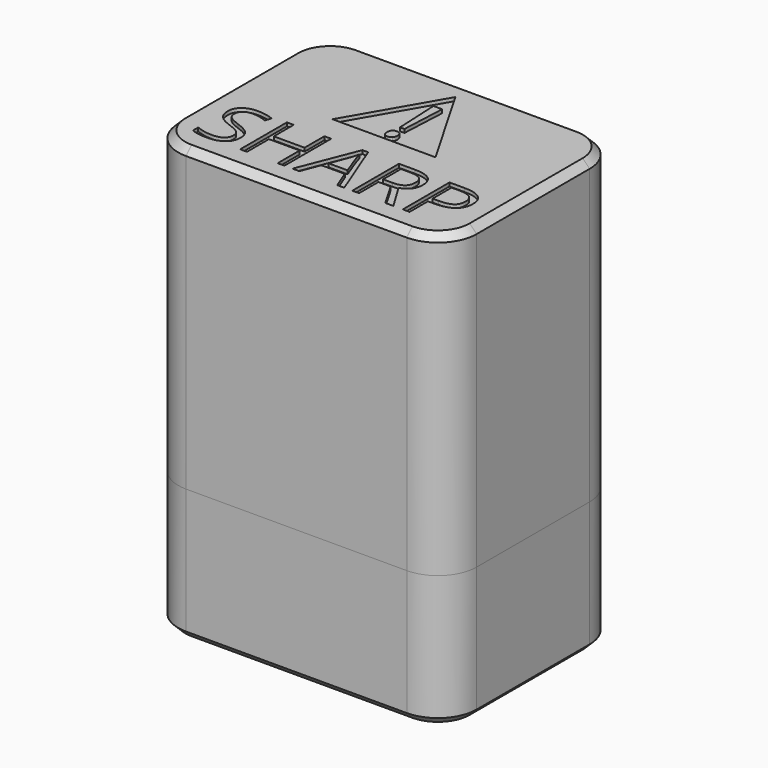
from build123d import *

# Parameters (mm, degrees)
F1_W          = 22
F1_H          = 43
F2_DEPTH      = 0.5
F4_DEPTH      = 37
F5_T          = 1.6
F7_DEPTH      = 15
F9_DEPTH      = 32
F11_DEPTH     = 2
F12_SIZE      = 0.8
F12_2_SIZE    = 0.8
F13_TEXT_SIZE = 9.2601952331
F14_DEPTH     = 0.4


# Not quite as in the source:
# - Text() gives the source's letters only with a copy of the font that has no kerning and outlines rounded to 1/6400 em; it was checked with that copy


with BuildPart() as f2:
    # F1 (on Front) → F2 (new body)
    with BuildSketch(Plane.XZ):
        with Locations((0, 21.5)):
            Rectangle(F1_W, F1_H)
    extrude(amount=F2_DEPTH)


with BuildPart() as f4:
    # F3 (on Top) → F4 (new body)
    with BuildSketch(Plane.XY):
        with BuildLine():
            Line((-12.5, -9), (12.5, -9))
            ThreePointArc((12.5, -9), (13.2071067812, -8.7071067812), (13.5, -8))
            Line((13.5, -8), (13.5, 8))
            ThreePointArc((13.5, 8), (13.2071067812, 8.7071067812), (12.5, 9))
            Line((12.5, 9), (-12.5, 9))
            ThreePointArc((-12.5, 9), (-13.2071067812, 8.7071067812), (-13.5, 8))
            Line((-13.5, 8), (-13.5, -8))
            ThreePointArc((-13.5, -8), (-13.2071067812, -8.7071067812), (-12.5, -9))
        make_face()
    extrude(amount=F4_DEPTH)

    # F5
    f5_openings = [f4.faces().sort_by_distance(p)[0] for p in [
        (0, 0, 37),
    ]]
    offset(amount=F5_T, openings=f5_openings, kind=Kind.INTERSECTION)

    # F6 (on face) → F7 (join)
    with BuildSketch(Plane(origin=(0, 0, -1.6), x_dir=(1, 0, 0), z_dir=(0, 0, -1))):
        with BuildLine():
            Line((-12.5, -12.4), (12.5, -12.4))
            ThreePointArc((12.5, -12.4), (15.6112698372, -11.1112698372), (16.9, -8))
            Line((16.9, -8), (16.9, 8))
            ThreePointArc((16.9, 8), (15.6112698372, 11.1112698372), (12.5, 12.4))
            Line((12.5, 12.4), (-12.5, 12.4))
            ThreePointArc((-12.5, 12.4), (-15.6112698372, 11.1112698372), (-16.9, 8))
            Line((-16.9, 8), (-16.9, -8))
            ThreePointArc((-16.9, -8), (-15.6112698372, -11.1112698372), (-12.5, -12.4))
        make_face()
        with BuildLine():
            Line((12.5, -10.6), (-12.5, -10.6))
            ThreePointArc((-12.5, -10.6), (-14.3384776311, -9.8384776311), (-15.1, -8))
            Line((-15.1, -8), (-15.1, 8))
            ThreePointArc((-15.1, 8), (-14.3384776311, 9.8384776311), (-12.5, 10.6))
            Line((-12.5, 10.6), (12.5, 10.6))
            ThreePointArc((12.5, 10.6), (14.3384776311, 9.8384776311), (15.1, 8))
            Line((15.1, 8), (15.1, -8))
            ThreePointArc((15.1, -8), (14.3384776311, -9.8384776311), (12.5, -10.6))
        make_face(mode=Mode.SUBTRACT)
    extrude(amount=-F7_DEPTH)

    # F12#2
    f12_2_edges = [f4.edges().sort_by_distance(p)[0] for p in [
        (16.9, 0, -1.6),
    ]]
    chamfer(f12_2_edges, length=F12_2_SIZE)


with BuildPart() as f9:
    # F8 (on face) → F9 (new body)
    with BuildSketch(Plane.XY.offset(13.4)):
        with BuildLine():
            Line((-12.5, -12.4), (12.5, -12.4))
            ThreePointArc((12.5, -12.4), (15.6112698372, -11.1112698372), (16.9, -8))
            Line((16.9, -8), (16.9, 8))
            ThreePointArc((16.9, 8), (15.6112698372, 11.1112698372), (12.5, 12.4))
            Line((12.5, 12.4), (-12.5, 12.4))
            ThreePointArc((-12.5, 12.4), (-15.6112698372, 11.1112698372), (-16.9, 8))
            Line((-16.9, 8), (-16.9, -8))
            ThreePointArc((-16.9, -8), (-15.6112698372, -11.1112698372), (-12.5, -12.4))
        make_face()
        with BuildLine():
            Line((12.5, -10.8), (-12.5, -10.8))
            ThreePointArc((-12.5, -10.8), (-14.4798989873, -9.9798989873), (-15.3, -8))
            Line((-15.3, -8), (-15.3, 8))
            ThreePointArc((-15.3, 8), (-14.4798989873, 9.9798989873), (-12.5, 10.8))
            Line((-12.5, 10.8), (12.5, 10.8))
            ThreePointArc((12.5, 10.8), (14.4798989873, 9.9798989873), (15.3, 8))
            Line((15.3, 8), (15.3, -8))
            ThreePointArc((15.3, -8), (14.4798989873, -9.9798989873), (12.5, -10.8))
        make_face(mode=Mode.SUBTRACT)
    extrude(amount=F9_DEPTH)

    # F10 (on face) → F11 (join)
    with BuildSketch(Plane.XY.offset(45.4)):
        with BuildLine():
            ThreePointArc((-16.9, -8), (-15.6112698372, -11.1112698372), (-12.5, -12.4))
            Line((-12.5, -12.4), (12.5, -12.4))
            ThreePointArc((12.5, -12.4), (15.6112698372, -11.1112698372), (16.9, -8))
            Line((16.9, -8), (16.9, 8))
            ThreePointArc((16.9, 8), (15.6112698372, 11.1112698372), (12.5, 12.4))
            Line((12.5, 12.4), (-12.5, 12.4))
            ThreePointArc((-12.5, 12.4), (-15.6112698372, 11.1112698372), (-16.9, 8))
            Line((-16.9, 8), (-16.9, -8))
        make_face()
    extrude(amount=F11_DEPTH)

    # F12
    f12_edges = [f9.edges().sort_by_distance(p)[0] for p in [
        (16.9, 0, 47.4),
    ]]
    chamfer(f12_edges, length=F12_SIZE)

    # F13 (on face) → F14 (cut)
    with BuildSketch(Plane.XY.offset(47.4)):
        Polygon((5.8312377188, 0), (0, 10.1), (-5.8312377188, 0), align=None)
        with BuildLine():
            add(Edge.make_bspline(
                [(-0.365185636, 0.6114120511), (-0.527236762, 0.7612903226), (-0.527236762, 1.1036518564)],
                knots=[0, 0, 0, 1, 1, 1], degree=2))
            add(Edge.make_bspline(
                [(-0.527236762, 1.1036518564), (-0.527236762, 1.7503347535), (0.0433657943, 1.7503347535)],
                knots=[0, 0, 0, 1, 1, 1], degree=2))
            add(Edge.make_bspline(
                [(0.0433657943, 1.7503347535), (0.3187766281, 1.7503347535), (0.4686548996, 1.5844796105)],
                knots=[0, 0, 0, 1, 1, 1], degree=2))
            add(Edge.make_bspline(
                [(0.4686548996, 1.5844796105), (0.618533171, 1.4186244674), (0.618533171, 1.1036518564)],
                knots=[0, 0, 0, 1, 1, 1], degree=2))
            add(Edge.make_bspline(
                [(0.618533171, 1.1036518564), (0.618533171, 0.799330493), (0.4663724893, 0.6304321363)],
                knots=[0, 0, 0, 1, 1, 1], degree=2))
            add(Edge.make_bspline(
                [(0.4663724893, 0.6304321363), (0.3142118077, 0.4615337797), (0.0433657943, 0.4615337797)],
                knots=[0, 0, 0, 1, 1, 1], degree=2))
            add(Edge.make_bspline(
                [(0.0433657943, 0.4615337797), (-0.20313451, 0.4615337797), (-0.365185636, 0.6114120511)],
                knots=[0, 0, 0, 1, 1, 1], degree=2))
        make_face(mode=Mode.SUBTRACT)
        Polygon((0.5424528302, 7.552221546), (0.3005173463, 2.5157029823), (-0.1985696896, 2.5157029823), (-0.4420267803, 7.552221546), align=None, mode=Mode.SUBTRACT)
        with Locations((-14.6, -9.6)):
            Text('SHARP', F13_TEXT_SIZE, font='Open Sans', text_align=(TextAlign.LEFT, TextAlign.BOTTOM))
    extrude(amount=-F14_DEPTH, mode=Mode.SUBTRACT)


solid = Compound([f2.part, f4.part, f9.part])
